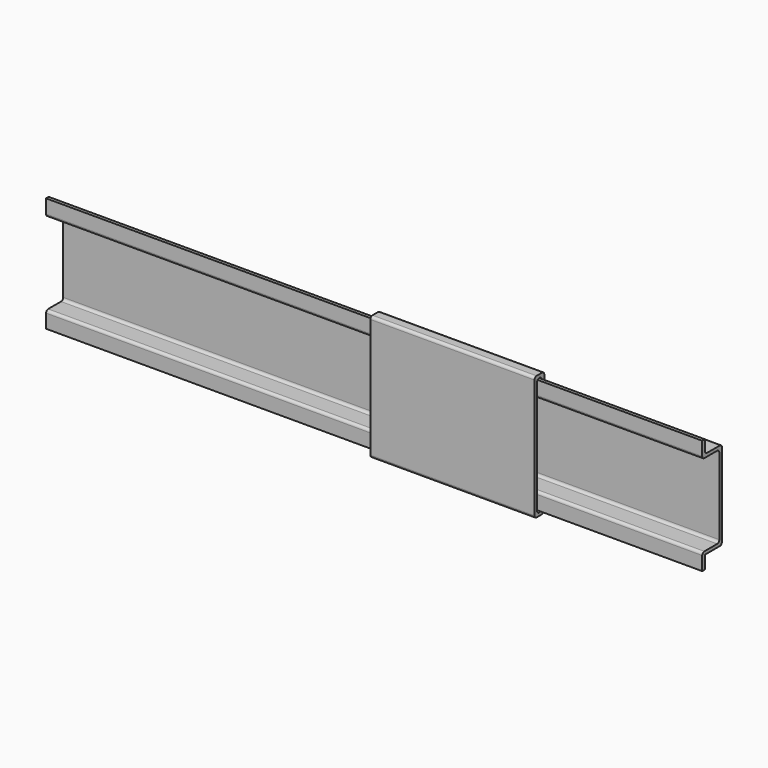
from build123d import *

# Parameters (mm, degrees)
F1_DEPTH    = 100
F2_R        = 0.8
F3_DEPTH    = 50
F4_T1_DEPTH = 50
F4_T3_DEPTH = 54


# Not quite as in the source:
# - a fillet or chamfer that OpenCascade refuses, or shapes differently, is made with other operations: its cross-section is extruded or revolved along the edge and cut away or added


with BuildPart() as f1:
    # F0 (on Right) → F1 (new body, symmetric)
    with BuildSketch(Plane.YZ):
        Polygon((1, 16.6007670015), (0, 16.6007670015), (0, 11.6007670015), (6.5, 11.6007670015), (6.5, -13.3992329985), (0, -13.3992329985), (0, -18.3992329985), (1, -18.3992329985), (1, -14.3992329985), (7.5, -14.3992329985), (7.5, 12.6007670015), (1, 12.6007670015), align=None)
    extrude(amount=F1_DEPTH, both=True)

    # F2
    f2_edges = [f1.edges().sort_by_distance(p)[0] for p in [
        (0, 1, 12.600767),
        (0, 0, 11.600767),
        (0, 7.5, 12.600767),
        (0, 6.5, 11.600767),
        (0, 7.5, -14.399233),
        (0, 0, -13.399233),
        (0, 6.5, -13.399233),
    ]]
    fillet(f2_edges, radius=F2_R)


with BuildPart() as f3:
    # F0 (on Right) → F3 (new body)
    with BuildSketch(Plane.YZ):
        Polygon((1.3245146256, 17.0073675215), (1.3245146256, 14.6007670015), (2.3245146256, 14.6007670015), (2.3245146256, 18.0073675215), (-1.4227514728, 18.0073675215), (-1.4227514728, -19.9926324785), (2.0886021191, -19.9926324785), (2.0886021191, -15.9926324785), (1.0886021191, -15.9926324785), (1.0886021191, -19.1249549389), (-0.4227514728, -19.1249549389), (-0.4227514728, 17.0073675215), align=None)
    extrude(amount=F3_DEPTH)

    # F4: fillet of radius 0.8 on 8 edges, made by hand

    # F4_s2 → F4_t1 (join)
    with BuildSketch(Plane.YZ):
        with BuildLine():
            ThreePointArc((-0.4227514728, 16.2073675215), (-0.1884368977, 16.7730529465), (0.3772485272, 17.0073675215))
            Line((0.3772485272, 17.0073675215), (-0.4227514728, 17.0073675215))
            Line((-0.4227514728, 17.0073675215), (-0.4227514728, 16.2073675215))
        make_face()
        with BuildLine():
            ThreePointArc((0.5245146256, 17.0073675215), (1.0902000505, 16.7730529465), (1.3245146256, 16.2073675215))
            Line((1.3245146256, 16.2073675215), (1.3245146256, 17.0073675215))
            Line((1.3245146256, 17.0073675215), (0.5245146256, 17.0073675215))
        make_face()
        with BuildLine():
            ThreePointArc((0.3772485272, -19.1249549389), (-0.1884368977, -18.8906403638), (-0.4227514728, -18.3249549389))
            Line((-0.4227514728, -18.3249549389), (-0.4227514728, -19.1249549389))
            Line((-0.4227514728, -19.1249549389), (0.3772485272, -19.1249549389))
        make_face()
        with BuildLine():
            ThreePointArc((1.0886021191, -18.3249549389), (0.8542875441, -18.8906403638), (0.2886021191, -19.1249549389))
            Line((0.2886021191, -19.1249549389), (1.0886021191, -19.1249549389))
            Line((1.0886021191, -19.1249549389), (1.0886021191, -18.3249549389))
        make_face()
    extrude(amount=F4_T1_DEPTH)

    # F4_s4 → F4_t3 (cut)
    with BuildSketch(Plane.YZ.offset(-2)):
        with BuildLine():
            ThreePointArc((-1.4227514728, 17.2073675215), (-1.1884368977, 17.7730529465), (-0.6227514728, 18.0073675215))
            Line((-0.6227514728, 18.0073675215), (-1.4227514728, 18.0073675215))
            Line((-1.4227514728, 18.0073675215), (-1.4227514728, 17.2073675215))
        make_face()
        with BuildLine():
            ThreePointArc((2.3245146256, 17.2073675215), (2.0902000505, 17.7730529465), (1.5245146256, 18.0073675215))
            Line((1.5245146256, 18.0073675215), (2.3245146256, 18.0073675215))
            Line((2.3245146256, 18.0073675215), (2.3245146256, 17.2073675215))
        make_face()
        with BuildLine():
            ThreePointArc((-0.6227514728, -19.9926324785), (-1.1884368977, -19.7583179034), (-1.4227514728, -19.1926324785))
            Line((-1.4227514728, -19.1926324785), (-1.4227514728, -19.9926324785))
            Line((-1.4227514728, -19.9926324785), (-0.6227514728, -19.9926324785))
        make_face()
        with BuildLine():
            ThreePointArc((2.0886021191, -19.1926324785), (1.8542875441, -19.7583179034), (1.2886021191, -19.9926324785))
            Line((1.2886021191, -19.9926324785), (2.0886021191, -19.9926324785))
            Line((2.0886021191, -19.9926324785), (2.0886021191, -19.1926324785))
        make_face()
    extrude(amount=F4_T3_DEPTH, mode=Mode.SUBTRACT)


solid = Compound([f1.part, f3.part])
